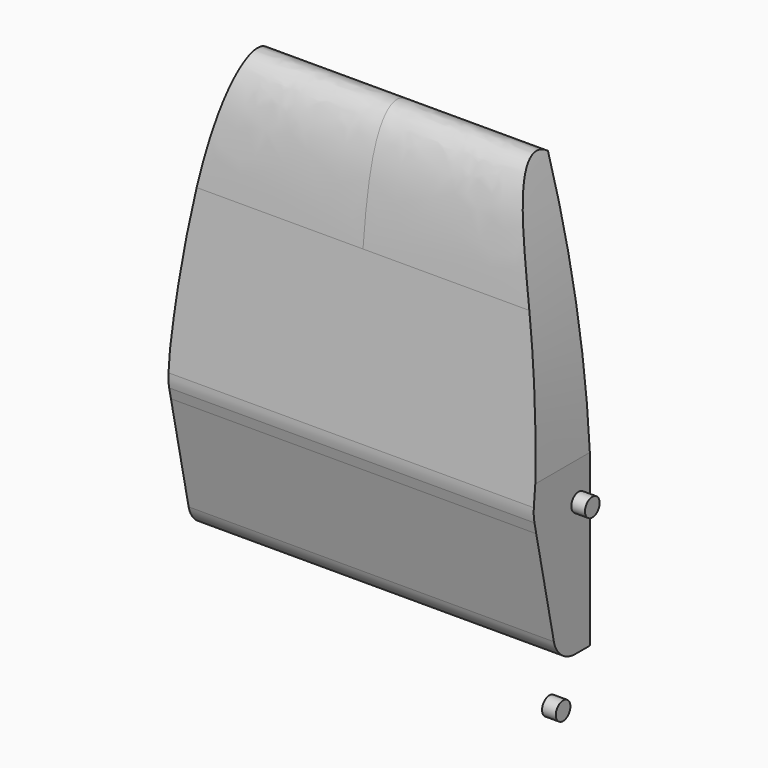
from build123d import *

# Parameters (mm, degrees)
F1_DEPTH = 200
F4_DEPTH = 100
F2_R     = 10
F5_DEPTH = 15


# Not quite as in the source:
# - a feature of the source that left no trace in its solid (it failed there, or was rolled back) is left out
# - a pattern or mirror of a feature is missing from the dataset's text; its kind, count and spacing are read off the source's solid
# - a feature names something its author has since deleted; it is built from what else it names


with BuildPart() as f1:
    # F0 (on Right) → F1 (new body, symmetric)
    with BuildSketch(Plane.YZ):
        with BuildLine():
            Line((55.3607484261, 155), (55.3607484261, 617.148949861))
            add(Edge.make_bspline(
                [(-5.1356334681, 496.9733605758), (-1.2527495457, 539.6434441922), (10.2970207059, 611.4394103819), (39.6879700651, 628.5664346662), (55.3607484261, 617.148949861)],
                knots=[0.7199137006, 0.7199137006, 0.7199137006, 0.7199137006, 0.8642094186, 0.999917509, 0.999917509, 0.999917509, 0.999917509], degree=3))
            add(Edge.make_bspline(
                [(-18.0039532914, 292.7610744649), (-17.7275211213, 295.6500029476), (-12.1238736433, 356.7123411708), (-10.7984274846, 434.7433534423), (-5.1356334681, 496.9733605758)],
                knots=[0.4988819934, 0.4988819934, 0.4988819934, 0.4988819934, 0.5094729702, 0.7199137006, 0.7199137006, 0.7199137006, 0.7199137006], degree=3))
            Line((-18.0039532914, 292.7610744649), (6.1743674758, 178.7750072777))
            ThreePointArc((6.1743674758, 178.7750072777), (16.6368991944, 161.6895969397), (35.5214195528, 155))
            Line((35.5214195528, 155), (55.3607484261, 155))
        make_face()
        with BuildLine():
            add(Edge.make_bspline(
                [(-18.0039532914, 292.7610744649), (-17.7275211213, 295.6500029476), (-12.1238736433, 356.7123411708), (-10.7984274846, 434.7433534423), (-5.1356334681, 496.9733605758)],
                knots=[0.4988819934, 0.4988819934, 0.4988819934, 0.4988819934, 0.5094729702, 0.7199137006, 0.7199137006, 0.7199137006, 0.7199137006], degree=3))
            Line((-5.1356334681, 496.9733605758), (-21.3186630339, 319.1335800048))
            ThreePointArc((-21.3186630339, 319.1335800048), (-21.4370021949, 311.6473714943), (-20.436154657, 304.2274236355))
            Line((-20.436154657, 304.2274236355), (-18.0039532914, 292.7610744649))
        make_face()
    extrude(amount=F1_DEPTH, both=True)

    # F3 (on Front) → F4 (cut, symmetric)
    with BuildSketch(Plane.XZ):
        with BuildLine():
            ThreePointArc((-200.4893869162, 330.5467367172), (-184.2445033895, 485.0446179169), (-148.4963000619, 636.2251639366))
            Line((-148.4963000619, 636.2251639366), (-242.7955716848, 636.2251639366))
            Line((-242.7955716848, 636.2251639366), (-242.7955716848, 330.5467367172))
            Line((-242.7955716848, 330.5467367172), (-200.4893869162, 330.5467367172))
        make_face()
    f4 = extrude(amount=F4_DEPTH, both=True, mode=Mode.SUBTRACT)

    # F4_copies: F4 across plane
    add(f4.mirror(Plane(origin=(0.000242, 0, 0), x_dir=(-1e-06, 0, 1), z_dir=(1, 0, 1e-06))), mode=Mode.SUBTRACT)

    # F2 (on face) → F5 (join)
    with BuildSketch(Plane.YZ.offset(200)):
        with Locations((40, 299.6807744877)):
            Circle(F2_R)
    extrude(amount=F5_DEPTH)


with BuildPart() as f5:
    # F2 (on face) → F5, piece 2 (new body)
    with BuildSketch(Plane.YZ.offset(200)):
        with Locations((0, 119.6807744877)):
            Circle(F2_R)
    extrude(amount=F5_DEPTH)


solid = Compound([f1.part, f5.part])
